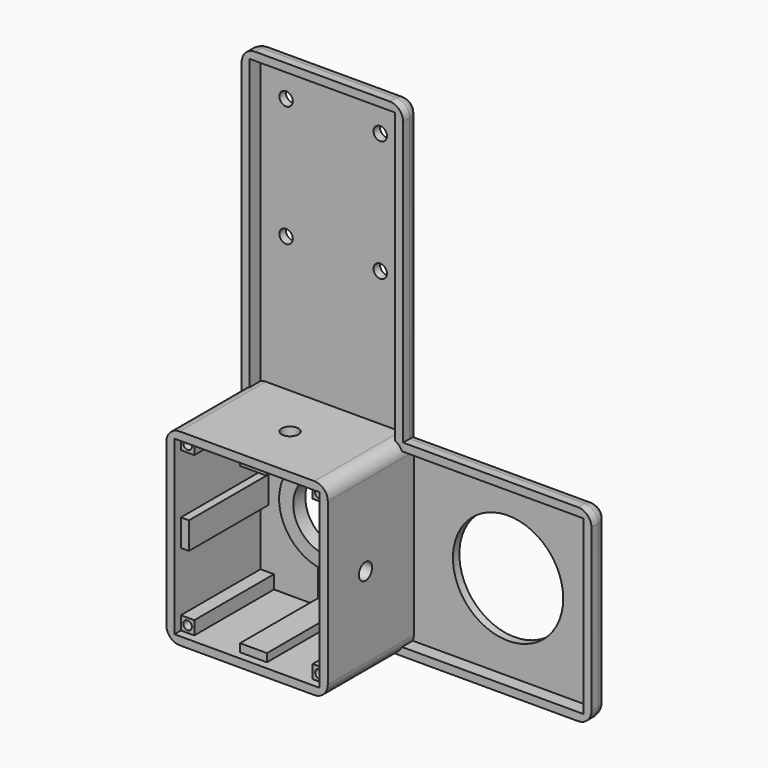
from build123d import *

# Parameters (mm, degrees)
F0_W          = 60
F0_H          = 180
F0_R          = 12.75
F0_R_2        = 2.5
F1_DEPTH      = 3
F2_R          = 18
F2_R_2        = 12.75
F3_DEPTH      = 2.6
F4_W          = 60
F4_H          = 70
F4_W_2        = 54
F4_H_2        = 64
F5_DEPTH      = 40
F6_W          = 5
F6_H          = 5
F6_W_2        = 10
F6_H_2        = 3
F6_W_3        = 3
F6_H_3        = 10
F7_DEPTH      = 37
F8_R          = 1.6
F9_DEPTH      = 28
F10_W         = 3
F10_H         = 70
F11_DEPTH     = 70
F13_R         = 20.5
F14_DEPTH     = 3
F16_DEPTH     = 5
F17_R         = 3.075
F18_DEPTH     = 6
F19_R         = 3.1
F20_DEPTH     = 6
F22_DEPTH     = 5
F23_R         = 5
F24_T1_DEPTH  = 47.5
F24_T3_DEPTH  = 50.5
F24_T5_DEPTH  = 15.5
F24_S9_W      = 5.1
F24_S9_H      = 5.1
F24_T10_DEPTH = 5.1
F24_S15_W     = 5.1
F24_S15_H     = 5.1
F24_T16_DEPTH = 5.1
F24_S21_W     = 5.1
F24_S21_H     = 5.1
F24_T22_DEPTH = 5.1
F24_S27_W     = 5.1
F24_S27_H     = 5.1
F24_T28_DEPTH = 5.1
F24_S33_W     = 5.1
F24_S33_H     = 5.1
F24_T34_DEPTH = 5.1
F24_T40_DEPTH = 60
F24_T46_DEPTH = 60
F24_T52_DEPTH = 60
F24_T58_DEPTH = 60


# Not quite as in the source:
# - a fillet or chamfer that OpenCascade refuses, or shapes differently, is made with other operations: its cross-section is extruded or revolved along the edge and cut away or added


with BuildPart() as f1:
    # F0 (on Front) → F1 (new body)
    with BuildSketch(Plane.XZ):
        Rectangle(F0_W, F0_H)
        with Locations((0, -55)):
            Circle(F0_R, mode=Mode.SUBTRACT)
        with Locations((-17.5, 30)):
            Circle(F0_R_2, mode=Mode.SUBTRACT)
        with Locations((-17.5, 75)):
            Circle(F0_R_2, mode=Mode.SUBTRACT)
        with Locations((17.5, 30)):
            Circle(F0_R_2, mode=Mode.SUBTRACT)
        with Locations((17.5, 75)):
            Circle(F0_R_2, mode=Mode.SUBTRACT)
    extrude(amount=-F1_DEPTH)

    # F2 (on face) → F3 (join)
    with BuildSketch(Plane.XZ):
        with Locations((0, -55)):
            Circle(F2_R)
        with Locations((0, -55)):
            Circle(F2_R_2, mode=Mode.SUBTRACT)
    extrude(amount=F3_DEPTH)

    # F4 (on face) → F5 (join)
    with BuildSketch(Plane.XZ):
        with Locations((0, -55)):
            Rectangle(F4_W, F4_H)
        with Locations((0, -55)):
            Rectangle(F4_W_2, F4_H_2, mode=Mode.SUBTRACT)
    extrude(amount=F5_DEPTH)

    # F6 (on face) → F7 (join)
    with BuildSketch(Plane.XZ):
        with Locations((-24.5, -25.5)):
            Rectangle(F6_W, F6_H)
        with Locations((0, -24.5)):
            Rectangle(F6_W_2, F6_H_2)
        with Locations((24.5, -25.5)):
            Rectangle(F6_W, F6_H)
        with Locations((25.5, -55)):
            Rectangle(F6_W_3, F6_H_3)
        with Locations((-25.5, -55)):
            Rectangle(F6_W_3, F6_H_3)
        with Locations((24.5, -84.5)):
            Rectangle(F6_W, F6_H)
        with Locations((0, -85.5)):
            Rectangle(F6_W_2, F6_H_2)
        with Locations((-24.5, -84.5)):
            Rectangle(F6_W, F6_H)
    extrude(amount=F7_DEPTH)

    # F8 (on face) → F9 (cut)
    with BuildSketch(Plane.XZ.offset(37)):
        with Locations((24.5, -25.5)):
            Circle(F8_R)
        with Locations((-24.5, -25.5)):
            Circle(F8_R)
        with Locations((24.5, -84.5)):
            Circle(F8_R)
        with Locations((-24.5, -84.5)):
            Circle(F8_R)
    extrude(amount=-F9_DEPTH, mode=Mode.SUBTRACT)

    # F10 (on face) → F11 (join)
    with BuildSketch(Plane.YZ.offset(30)):
        with Locations((1.5, -55)):
            Rectangle(F10_W, F10_H)
    extrude(amount=F11_DEPTH)

    # F13 (on face) → F14 (cut, through all)
    with BuildSketch(Plane.XZ):
        with Locations((65, -55)):
            Circle(F13_R)
    extrude(amount=-F14_DEPTH, mode=Mode.SUBTRACT)

    # F15 (on face) → F16 (join)
    with BuildSketch(Plane.XZ):
        Polygon((100, -20), (30, -20), (30, -23), (97, -23), (97, -87), (30, -87), (30, -90), (100, -90), (100, -87), (100, -23), align=None)
    extrude(amount=F16_DEPTH)

    # F17 (on face) → F18 (cut, through all)
    with BuildSketch(Plane.YZ.offset(30)):
        with Locations((-22.5, -55)):
            Circle(F17_R)
    extrude(amount=-F18_DEPTH, mode=Mode.SUBTRACT)

    # F19 (on face) → F20 (cut, through all)
    with BuildSketch(Plane.XY.offset(-20)):
        with Locations((0, -20)):
            Circle(F19_R)
    extrude(amount=-F20_DEPTH, mode=Mode.SUBTRACT)

    # F21 (on face) → F22 (join)
    with BuildSketch(Plane.XZ):
        Polygon((30, -20), (30, 90), (27, 90), (21.6846410185, 90), (-27, 90), (-30, 90), (-30, -20), (-27, -20), (-27, 87), (27, 87), (27, -20), align=None)
    extrude(amount=F22_DEPTH)

    # F23
    f23_edges = [f1.edges().sort_by_distance(p)[0] for p in [
        (35, 3, -90),
        (-30, 3, 0),
        (0, 3, 90),
        (30, 3, 35),
        (65, 3, -20),
        (100, 3, -55),
    ]]
    fillet(f23_edges, radius=F23_R)

    # F24: fillet of radius 5 on 8 edges, made by hand

    # F24_s2 → F24_t1 (cut)
    with BuildSketch(Plane.XZ.offset(5)):
        with BuildLine():
            ThreePointArc((30, -25), (28.5355339059, -21.4644660941), (25, -20))
            Line((25, -20), (30, -20))
            Line((30, -20), (30, -25))
        make_face()
        with BuildLine():
            ThreePointArc((-30, -25), (-28.5355339059, -21.4644660941), (-25, -20))
            Line((-25, -20), (-30, -20))
            Line((-30, -20), (-30, -25))
        make_face()
        with BuildLine():
            ThreePointArc((25, -90), (28.5355339059, -88.5355339059), (30, -85))
            Line((30, -85), (30, -90))
            Line((30, -90), (25, -90))
        make_face()
    extrude(amount=F24_T1_DEPTH, mode=Mode.SUBTRACT)

    # F24_s4 → F24_t3 (cut)
    with BuildSketch(Plane.XZ.offset(2)):
        with BuildLine():
            ThreePointArc((-25, -90), (-28.5355339059, -88.5355339059), (-30, -85))
            Line((-30, -85), (-30, -90))
            Line((-30, -90), (-25, -90))
        make_face()
    extrude(amount=F24_T3_DEPTH, mode=Mode.SUBTRACT)

    # F24_s6 → F24_t5 (cut)
    with BuildSketch(Plane.XZ.offset(2)):
        with BuildLine():
            ThreePointArc((100, -25), (98.5355339059, -21.4644660941), (95, -20))
            Line((95, -20), (100, -20))
            Line((100, -20), (100, -25))
        make_face()
        with BuildLine():
            ThreePointArc((95, -90), (98.5355339059, -88.5355339059), (100, -85))
            Line((100, -85), (100, -90))
            Line((100, -90), (95, -90))
        make_face()
        with BuildLine():
            ThreePointArc((25, 90), (28.5355339059, 88.5355339059), (30, 85))
            Line((30, 85), (30, 90))
            Line((30, 90), (25, 90))
        make_face()
        with BuildLine():
            ThreePointArc((-30, 85), (-28.5355339059, 88.5355339059), (-25, 90))
            Line((-25, 90), (-30, 90))
            Line((-30, 90), (-30, 85))
        make_face()
    extrude(amount=F24_T5_DEPTH, mode=Mode.SUBTRACT)


with BuildPart() as f24_tool8:
    # F24_s9 → F24_t10 (new body)
    with BuildSketch(Plane.YZ.offset(-25)):
        with Locations((0.55, 87.55)):
            Rectangle(F24_S9_W, F24_S9_H)
    extrude(amount=-F24_T10_DEPTH)

    # F24_s11 → F24_t12 (revolve, cut)
    with BuildSketch(Plane(origin=(-25, -2, 85), x_dir=(0, -0.7071067812, -0.7071067812), z_dir=(0, 0.7071067812, -0.7071067812))):
        with BuildLine():
            ThreePointArc((0, -5), (5, 0), (0, 5))
            Line((0, 5), (0, -5))
        make_face()
    revolve(axis=Axis((-25, -2, 85), (-1, 0, 0)), mode=Mode.SUBTRACT)


with BuildPart() as f1_1:
    add(f1.part)

    # F24_t7: cut F24_tool8
    add(f24_tool8.part, mode=Mode.SUBTRACT)


with BuildPart() as f24_tool14:
    # F24_s15 → F24_t16 (new body)
    with BuildSketch(Plane.XY.offset(85)):
        with Locations((27.55, 0.55)):
            Rectangle(F24_S15_W, F24_S15_H)
    extrude(amount=F24_T16_DEPTH)

    # F24_s17 → F24_t18 (revolve, cut)
    with BuildSketch(Plane(origin=(25, -2, 85), x_dir=(-0.7071067812, -0.7071067812, 0), z_dir=(-0.7071067812, 0.7071067812, 0))):
        with BuildLine():
            ThreePointArc((0, -5), (5, 0), (0, 5))
            Line((0, 5), (0, -5))
        make_face()
    revolve(axis=Axis((25, -2, 85), (0, 0, 1)), mode=Mode.SUBTRACT)


with BuildPart() as f1_2:
    add(f1_1.part)

    # F24_t13: cut F24_tool14
    add(f24_tool14.part, mode=Mode.SUBTRACT)


with BuildPart() as f24_tool20:
    # F24_s21 → F24_t22 (new body)
    with BuildSketch(Plane.XY.offset(-85)):
        with Locations((97.55, 0.55)):
            Rectangle(F24_S21_W, F24_S21_H)
    extrude(amount=-F24_T22_DEPTH)

    # F24_s23 → F24_t24 (revolve, cut)
    with BuildSketch(Plane(origin=(95, -2, -85), x_dir=(-0.7071067812, -0.7071067812, 0), z_dir=(0.7071067812, -0.7071067812, 0))):
        with BuildLine():
            ThreePointArc((0, -5), (5, 0), (0, 5))
            Line((0, 5), (0, -5))
        make_face()
    revolve(axis=Axis((95, -2, -85), (0, 0, -1)), mode=Mode.SUBTRACT)


with BuildPart() as f1_3:
    add(f1_2.part)

    # F24_t19: cut F24_tool20
    add(f24_tool20.part, mode=Mode.SUBTRACT)


with BuildPart() as f24_tool26:
    # F24_s27 → F24_t28 (new body)
    with BuildSketch(Plane.YZ.offset(95)):
        with Locations((0.55, -22.45)):
            Rectangle(F24_S27_W, F24_S27_H)
    extrude(amount=F24_T28_DEPTH)

    # F24_s29 → F24_t30 (revolve, cut)
    with BuildSketch(Plane(origin=(95, -2, -25), x_dir=(0, -0.7071067812, -0.7071067812), z_dir=(0, -0.7071067812, 0.7071067812))):
        with BuildLine():
            ThreePointArc((0, -5), (5, 0), (0, 5))
            Line((0, 5), (0, -5))
        make_face()
    revolve(axis=Axis((95, -2, -25), (1, 0, 0)), mode=Mode.SUBTRACT)


with BuildPart() as f1_4:
    add(f1_3.part)

    # F24_t25: cut F24_tool26
    add(f24_tool26.part, mode=Mode.SUBTRACT)


with BuildPart() as f24_tool32:
    # F24_s33 → F24_t34 (new body)
    with BuildSketch(Plane.XY.offset(-85)):
        with Locations((-27.55, 0.55)):
            Rectangle(F24_S33_W, F24_S33_H)
    extrude(amount=-F24_T34_DEPTH)

    # F24_s35 → F24_t36 (revolve, cut)
    with BuildSketch(Plane(origin=(-25, -2, -85), x_dir=(0.7071067812, -0.7071067812, 0), z_dir=(0.7071067812, 0.7071067812, 0))):
        with BuildLine():
            ThreePointArc((0, -5), (5, 0), (0, 5))
            Line((0, 5), (0, -5))
        make_face()
    revolve(axis=Axis((-25, -2, -85), (0, 0, -1)), mode=Mode.SUBTRACT)


with BuildPart() as f1_5:
    add(f1_4.part)

    # F24_t31: cut F24_tool32
    add(f24_tool32.part, mode=Mode.SUBTRACT)


with BuildPart() as f24_tool38:
    # F24_s39 → F24_t40 (new body)
    with BuildSketch(Plane.XZ.offset(-7.5)):
        with BuildLine():
            ThreePointArc((30, -25), (28.5355339059, -21.4644660941), (25, -20))
            Line((25, -20), (30, -20))
            Line((30, -20), (30, -25))
        make_face()
    extrude(amount=F24_T40_DEPTH)

    split(bisect_by=Plane.XY.offset(-23), keep=Keep.BOTTOM)

    split(bisect_by=Plane.XZ, keep=Keep.TOP)


with BuildPart() as f1_6:
    add(f1_5.part)

    # F24_t37: cut F24_tool38
    add(f24_tool38.part, mode=Mode.SUBTRACT)


with BuildPart() as f24_tool44:
    # F24_s45 → F24_t46 (new body)
    with BuildSketch(Plane.XZ.offset(-7.5)):
        with BuildLine():
            ThreePointArc((30, -25), (28.5355339059, -21.4644660941), (25, -20))
            Line((25, -20), (30, -20))
            Line((30, -20), (30, -25))
        make_face()
    extrude(amount=F24_T46_DEPTH)

    split(bisect_by=Plane.XZ, keep=Keep.TOP)

    split(bisect_by=Plane.YZ.offset(27), keep=Keep.BOTTOM)


with BuildPart() as f1_7:
    add(f1_6.part)

    # F24_t43: cut F24_tool44
    add(f24_tool44.part, mode=Mode.SUBTRACT)


with BuildPart() as f24_tool50:
    # F24_s51 → F24_t52 (new body)
    with BuildSketch(Plane.XZ.offset(-7.5)):
        with BuildLine():
            ThreePointArc((-30, -25), (-28.5355339059, -21.4644660941), (-25, -20))
            Line((-25, -20), (-30, -20))
            Line((-30, -20), (-30, -25))
        make_face()
    extrude(amount=F24_T52_DEPTH)

    split(bisect_by=Plane.XZ, keep=Keep.TOP)

    split(bisect_by=Plane.YZ.offset(-27), keep=Keep.TOP)


with BuildPart() as f1_8:
    add(f1_7.part)

    # F24_t49: cut F24_tool50
    add(f24_tool50.part, mode=Mode.SUBTRACT)


with BuildPart() as f24_tool56:
    # F24_s57 → F24_t58 (new body)
    with BuildSketch(Plane.XZ.offset(-7.5)):
        with BuildLine():
            ThreePointArc((25, -90), (28.5355339059, -88.5355339059), (30, -85))
            Line((30, -85), (30, -90))
            Line((30, -90), (25, -90))
        make_face()
    extrude(amount=F24_T58_DEPTH)

    split(bisect_by=Plane.XY.offset(-87), keep=Keep.TOP)

    split(bisect_by=Plane.XZ, keep=Keep.TOP)


with BuildPart() as f1_9:
    add(f1_8.part)

    # F24_t55: cut F24_tool56
    add(f24_tool56.part, mode=Mode.SUBTRACT)


solid = f1_9.part
